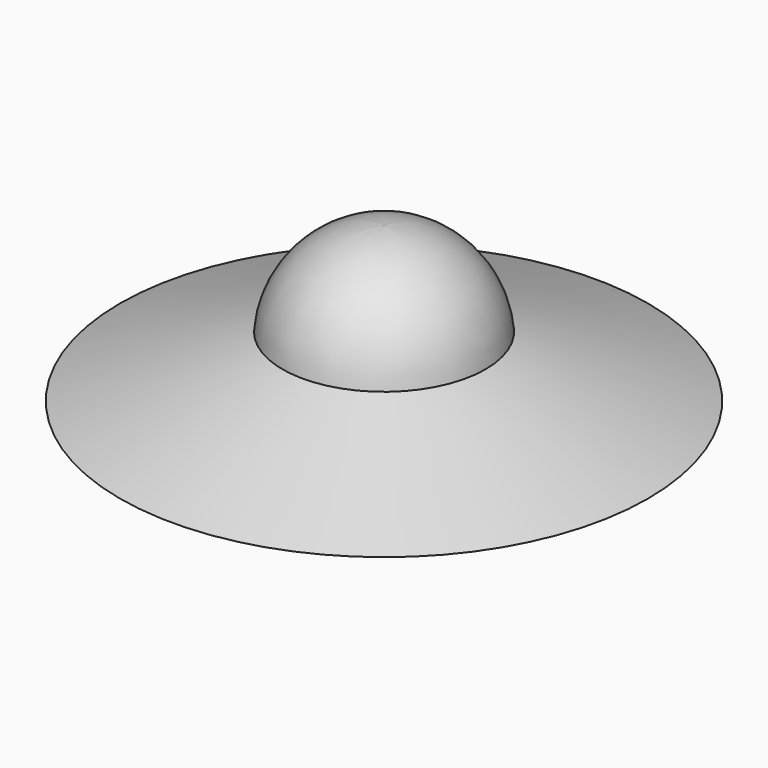
from build123d import *

# Parameters (mm, degrees)
F2_R      = 65
F3_R      = 25
F5_FACE_R = 65
F4_R      = 25
F7_DEPTH  = 23
F9_DEPTH  = 3


# Not quite as in the source:
# - a fillet or chamfer that OpenCascade refuses, or shapes differently, is made with other operations: its cross-section is extruded or revolved along the edge and cut away or added


with BuildPart() as f5:
    # F2 (on offset) → F5 section 0
    with BuildSketch(Plane.XY.offset(15)):
        Circle(F2_R)
    # F3 (on offset) → F5 section 1
    with BuildSketch(Plane.XY.offset(30)):
        Circle(F3_R)
    loft()

    # F5_face (on face) → F6 section 0
    with BuildSketch(Plane(origin=(0, 0, 15), x_dir=(1, 0, 0), z_dir=(0, 0, -1))):
        Circle(F5_FACE_R)
    # F4 (on Top) → F6 section 1
    with BuildSketch(Plane.XY):
        Circle(F4_R)
    loft()

    # F7 (add): a face of the model
    f7_faces = [f5.faces().sort_by_distance(p)[0] for p in [
        (0, 0, 30),
    ]]
    extrude(f7_faces, amount=F7_DEPTH)

    # F8: fillet of radius 25 on 1 edges, made by hand

    # F8_s1 → F8_t2 (revolve, cut)
    with BuildSketch(Plane.XZ):
        with BuildLine():
            ThreePointArc((25, 30), (17.0359533691, 46.3711730709), (0.0801284112, 53))
            Line((0.0801284112, 53), (25, 53))
            Line((25, 53), (25, 30))
        make_face()
    revolve(axis=Axis((0, 0, 53), (0, 0, 1)), mode=Mode.SUBTRACT)

    # F9 (add): a face of the model
    f9_faces = [f5.faces().sort_by_distance(p)[0] for p in [
        (0, 0, 0),
    ]]
    extrude(f9_faces, amount=F9_DEPTH)


solid = f5.part
